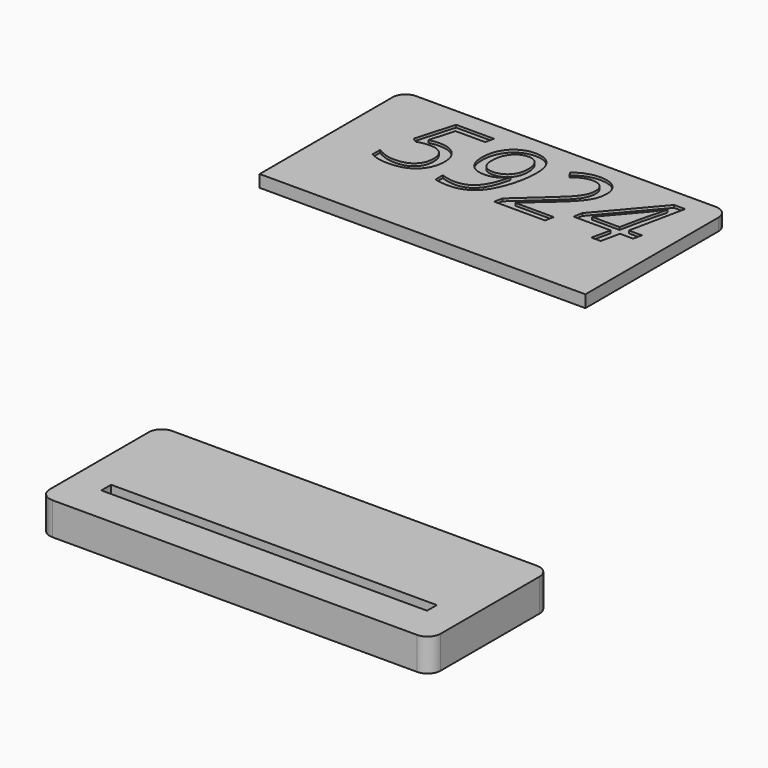
from build123d import *

# Parameters (mm, degrees)
F3_W         = 152.4
F3_H         = 58.42
F3_W_2       = 127
F3_H_2       = 4.7625
F4_DEPTH     = 12.7
F5_W         = 127
F5_H         = 4.7625
F5_W_2       = 35.6893126208
F5_H_2       = 5.08
F6_DEPTH     = 5.08
F7_R         = 5.08
F8_DEPTH     = 8.89
F9_W         = 127
F9_H         = 69.85
F10_DEPTH    = 4.7625
F9_TEXT_SIZE = 45.3111405174
F11_DEPTH    = 3.7625
F12_R        = 5.08
F13_DEPTH    = 3.302


# Not quite as in the source:
# - a length typed as a fraction of an inch, garbled in the dataset ("3 / 203.2 mm" for 3/8 in), is restored
# - a feature names something its author has since deleted; it is built from what else it names
# - Text() gives the source's letters only with a copy of the font that has no kerning and outlines rounded to 1/6400 em; it was checked with that copy


with BuildPart() as f4:
    # F3 (on Top) → F4 (new body)
    with BuildSketch(Plane.XY):
        with Locations((-9.5931086689, 18.5555488393)):
            Rectangle(F3_W, F3_H)
        with Locations((-9.5931086689, 6.0863080435)):
            Rectangle(F3_W_2, F3_H_2, mode=Mode.SUBTRACT)
    extrude(amount=F4_DEPTH)

    # F5 (on face) → F6 (cut)
    with BuildSketch(Plane(origin=(0, 0, 0), x_dir=(1, 0, 0), z_dir=(0, 0, -1))):
        Polygon((59.2411287415, -1.0063080435), (-78.4273460794, -1.0063080435), (-78.4273460794, -11.1663080435), (23.5518161207, -11.1663080435), (59.2411287415, -11.1663080435), align=None)
        with Locations((-9.5931086689, -6.0863080435)):
            Rectangle(F5_W, F5_H, mode=Mode.SUBTRACT)
        with Locations((41.3964724311, -13.7063080435)):
            Rectangle(F5_W_2, F5_H_2)
    extrude(amount=-F6_DEPTH, mode=Mode.SUBTRACT)

    # F7
    f7_edges = [f4.edges().sort_by_distance(p)[0] for p in [
        (-85.793109, -10.654451, 6.35),
        (66.606891, -10.654451, 6.35),
        (66.606891, 47.765549, 6.35),
        (-85.793109, 47.765549, 6.35),
    ]]
    fillet(f7_edges, radius=F7_R)

    # F5 (on face) → F8 (cut)
    with BuildSketch(Plane(origin=(0, 0, 0), x_dir=(1, 0, 0), z_dir=(0, 0, -1))):
        Polygon((59.2411287415, -41.7463080435), (59.2411287415, -16.2463080435), (23.5518161207, -16.2463080435), (10.8411287415, -16.2463080435), (10.8411287415, -27.1657891572), (10.8411287415, -30.3407891572), (10.8411287415, -41.7463080435), align=None)
    extrude(amount=-F8_DEPTH, mode=Mode.SUBTRACT)

    # F5 (on face) → F13 (cut)
    with BuildSketch(Plane(origin=(0, 0, 0), x_dir=(1, 0, 0), z_dir=(0, 0, -1))):
        Polygon((10.8411287415, -30.3407891572), (10.8411287415, -27.1657891572), (-11.5801747888, -27.1657891572), (-11.5801747888, -47.7655488393), (-8.4051747888, -47.7655488393), (-8.4051747888, -30.3407891572), align=None)
    extrude(amount=-F13_DEPTH, mode=Mode.SUBTRACT)


with BuildPart() as f10:
    # F9 (on Top) → F10 (new body)
    with BuildSketch(Plane.XY):
        with Locations((-111.8032857776, 243.5436563784)):
            Rectangle(F9_W, F9_H)
        with BuildLine():
            add(Edge.make_bspline(
                [(-149.1894343829, 258.2214627279), (-147.2637109109, 258.7312130587), (-145.118511602, 258.7312130587)],
                knots=[0, 0, 0, 1, 1, 1], degree=2))
            add(Edge.make_bspline(
                [(-145.118511602, 258.7312130587), (-141.0900680154, 258.7312130587), (-138.7147730711, 256.4196369058)],
                knots=[0, 0, 0, 1, 1, 1], degree=2))
            add(Edge.make_bspline(
                [(-138.7147730711, 256.4196369058), (-136.3394781268, 254.1080607528), (-136.3394781268, 250.1645755547)],
                knots=[0, 0, 0, 1, 1, 1], degree=2))
            add(Edge.make_bspline(
                [(-136.3394781268, 250.1645755547), (-136.3394781268, 246.6034031046), (-137.9536875077, 243.9059742707)],
                knots=[0, 0, 0, 1, 1, 1], degree=2))
            add(Edge.make_bspline(
                [(-137.9536875077, 243.9059742707), (-139.5678968887, 241.2085454368), (-142.4671018952, 239.8669108855)],
                knots=[0, 0, 0, 1, 1, 1], degree=2))
            add(Edge.make_bspline(
                [(-142.4671018952, 239.8669108855), (-145.3663069018, 238.5252763343), (-149.2814726371, 238.5252763343)],
                knots=[0, 0, 0, 1, 1, 1], degree=2))
            add(Edge.make_bspline(
                [(-149.2814726371, 238.5252763343), (-153.5506316577, 238.5252763343), (-156.5808141798, 240.2740031636)],
                knots=[0, 0, 0, 1, 1, 1], degree=2))
            Line((-156.5808141798, 240.2740031636), (-156.5808141798, 243.9059742707))
            add(Edge.make_bspline(
                [(-156.5808141798, 243.9059742707), (-152.9488430727, 241.6474971105), (-149.1894343829, 241.6474971105)],
                knots=[0, 0, 0, 1, 1, 1], degree=2))
            add(Edge.make_bspline(
                [(-149.1894343829, 241.6474971105), (-144.9627545565, 241.6474971105), (-142.5980794108, 243.7714568223)],
                knots=[0, 0, 0, 1, 1, 1], degree=2))
            add(Edge.make_bspline(
                [(-142.5980794108, 243.7714568223), (-140.233404265, 245.895416534), (-140.233404265, 249.7043842838)],
                knots=[0, 0, 0, 1, 1, 1], degree=2))
            add(Edge.make_bspline(
                [(-140.233404265, 249.7043842838), (-140.233404265, 252.4867715062), (-141.8582334445, 254.1151406185)],
                knots=[0, 0, 0, 1, 1, 1], degree=2))
            add(Edge.make_bspline(
                [(-141.8582334445, 254.1151406185), (-143.483062624, 255.7435097309), (-146.3787276977, 255.7435097309)],
                knots=[0, 0, 0, 1, 1, 1], degree=2))
            add(Edge.make_bspline(
                [(-146.3787276977, 255.7435097309), (-147.4407075536, 255.7435097309), (-148.5274669394, 255.5983724839)],
                knots=[0, 0, 0, 1, 1, 1], degree=2))
            add(Edge.make_bspline(
                [(-148.5274669394, 255.5983724839), (-149.6142263253, 255.4532352369), (-151.6036685886, 254.922245309)],
                knots=[0, 0, 0, 1, 1, 1], degree=2))
            Line((-151.6036685886, 254.922245309), (-153.2391175667, 256.1824614046))
            Line((-153.2391175667, 256.1824614046), (-148.8779202919, 271.3192142837))
            Line((-148.8779202919, 271.3192142837), (-134.1022405638, 271.3192142837))
            Line((-134.1022405638, 271.3192142837), (-134.8314667315, 267.9350384763))
            Line((-134.8314667315, 267.9350384763), (-146.3787276977, 267.9350384763))
            Line((-146.3787276977, 267.9350384763), (-149.1894343829, 258.2214627279))
        make_face(mode=Mode.SUBTRACT)
        with BuildLine():
            add(Edge.make_bspline(
                [(-111.9882800316, 269.2483535648), (-109.7899817299, 266.7173015749), (-109.7899817299, 261.8463539693)],
                knots=[0, 0, 0, 1, 1, 1], degree=2))
            add(Edge.make_bspline(
                [(-109.7899817299, 261.8463539693), (-109.7899817299, 257.5559553516), (-111.0289582284, 252.8549245229)],
                knots=[0, 0, 0, 1, 1, 1], degree=2))
            add(Edge.make_bspline(
                [(-111.0289582284, 252.8549245229), (-112.2679347269, 248.1538936942), (-114.289236386, 244.8900756038)],
                knots=[0, 0, 0, 1, 1, 1], degree=2))
            add(Edge.make_bspline(
                [(-114.289236386, 244.8900756038), (-116.310538045, 241.6262575134), (-119.1885034544, 240.0757669238)],
                knots=[0, 0, 0, 1, 1, 1], degree=2))
            add(Edge.make_bspline(
                [(-119.1885034544, 240.0757669238), (-122.0664688638, 238.5252763343), (-125.8683567479, 238.5252763343)],
                knots=[0, 0, 0, 1, 1, 1], degree=2))
            add(Edge.make_bspline(
                [(-125.8683567479, 238.5252763343), (-128.8772996728, 238.5252763343), (-131.2278150872, 239.2828219648)],
                knots=[0, 0, 0, 1, 1, 1], degree=2))
            Line((-131.2278150872, 239.2828219648), (-131.2278150872, 242.7802756235))
            add(Edge.make_bspline(
                [(-131.2278150872, 242.7802756235), (-128.2613513564, 241.7395353647), (-125.7833983594, 241.7395353647)],
                knots=[0, 0, 0, 1, 1, 1], degree=2))
            add(Edge.make_bspline(
                [(-125.7833983594, 241.7395353647), (-121.316003099, 241.7395353647), (-118.547775608, 244.8582162081)],
                knots=[0, 0, 0, 1, 1, 1], degree=2))
            add(Edge.make_bspline(
                [(-118.547775608, 244.8582162081), (-115.779548117, 247.9768970516), (-114.3635749759, 254.6107312179)],
                knots=[0, 0, 0, 1, 1, 1], degree=2))
            Line((-114.3635749759, 254.6107312179), (-114.5901306785, 254.6107312179))
            add(Edge.make_bspline(
                [(-114.5901306785, 254.6107312179), (-115.7158293257, 252.9540426428), (-117.5176551478, 251.9911809068)],
                knots=[0, 0, 0, 1, 1, 1], degree=2))
            add(Edge.make_bspline(
                [(-117.5176551478, 251.9911809068), (-119.31948097, 251.0283191708), (-121.5142393388, 251.0283191708)],
                knots=[0, 0, 0, 1, 1, 1], degree=2))
            add(Edge.make_bspline(
                [(-121.5142393388, 251.0283191708), (-125.2524084315, 251.0283191708), (-127.2878698219, 253.2089178082)],
                knots=[0, 0, 0, 1, 1, 1], degree=2))
            add(Edge.make_bspline(
                [(-127.2878698219, 253.2089178082), (-129.3233312123, 255.3895164456), (-129.3233312123, 259.5949566748)],
                knots=[0, 0, 0, 1, 1, 1], degree=2))
            add(Edge.make_bspline(
                [(-129.3233312123, 259.5949566748), (-129.3233312123, 262.9791324822), (-127.8967382726, 265.800458966)],
                knots=[0, 0, 0, 1, 1, 1], degree=2))
            add(Edge.make_bspline(
                [(-127.8967382726, 265.800458966), (-126.4701453329, 268.6217854498), (-123.9143138131, 270.2005955022)],
                knots=[0, 0, 0, 1, 1, 1], degree=2))
            add(Edge.make_bspline(
                [(-123.9143138131, 270.2005955022), (-121.3584822932, 271.7794055546), (-118.1725427256, 271.7794055546)],
                knots=[0, 0, 0, 1, 1, 1], degree=2))
            add(Edge.make_bspline(
                [(-118.1725427256, 271.7794055546), (-114.1865783332, 271.7794055546), (-111.9882800316, 269.2483535648)],
                knots=[0, 0, 0, 1, 1, 1], degree=2))
        make_face(mode=Mode.SUBTRACT)
        with BuildLine():
            Line((-87.6370819363, 242.3767232782), (-88.2813497155, 238.9713078737))
            Line((-88.2813497155, 238.9713078737), (-108.1686924833, 238.9713078737))
            Line((-108.1686924833, 238.9713078737), (-107.4890253755, 242.2209662327))
            Line((-107.4890253755, 242.2209662327), (-97.1949006392, 251.5168299045))
            add(Edge.make_bspline(
                [(-97.1949006392, 251.5168299045), (-94.9435033447, 253.5770708249), (-93.2938946353, 255.1346412802)],
                knots=[0, 0, 0, 1, 1, 1], degree=2))
            add(Edge.make_bspline(
                [(-93.2938946353, 255.1346412802), (-91.6442859258, 256.6922117355), (-90.5716862714, 258.0763254809)],
                knots=[0, 0, 0, 1, 1, 1], degree=2))
            add(Edge.make_bspline(
                [(-90.5716862714, 258.0763254809), (-89.4990866169, 259.4604392264), (-88.9787164876, 260.819773442)],
                knots=[0, 0, 0, 1, 1, 1], degree=2))
            add(Edge.make_bspline(
                [(-88.9787164876, 260.819773442), (-88.4583463582, 262.1791076575), (-88.4583463582, 263.8428760984)],
                knots=[0, 0, 0, 1, 1, 1], degree=2))
            add(Edge.make_bspline(
                [(-88.4583463582, 263.8428760984), (-88.4583463582, 266.0305546015), (-89.785821178, 267.3120102942)],
                knots=[0, 0, 0, 1, 1, 1], degree=2))
            add(Edge.make_bspline(
                [(-89.785821178, 267.3120102942), (-91.1132959979, 268.593465987), (-93.3930127552, 268.593465987)],
                knots=[0, 0, 0, 1, 1, 1], degree=2))
            add(Edge.make_bspline(
                [(-93.3930127552, 268.593465987), (-95.0992603903, 268.593465987), (-96.7240895698, 267.9633579392)],
                knots=[0, 0, 0, 1, 1, 1], degree=2))
            add(Edge.make_bspline(
                [(-96.7240895698, 267.9633579392), (-98.3489187493, 267.3332498913), (-100.3171214155, 265.8323183617)],
                knots=[0, 0, 0, 1, 1, 1], degree=2))
            Line((-100.3171214155, 265.8323183617), (-102.1295670362, 268.3739901501))
            add(Edge.make_bspline(
                [(-102.1295670362, 268.3739901501), (-97.9028872098, 271.7794055546), (-92.9965402756, 271.7794055546)],
                knots=[0, 0, 0, 1, 1, 1], degree=2))
            add(Edge.make_bspline(
                [(-92.9965402756, 271.7794055546), (-89.1026141374, 271.7794055546), (-86.8335171787, 269.8218226869)],
                knots=[0, 0, 0, 1, 1, 1], degree=2))
            add(Edge.make_bspline(
                [(-86.8335171787, 269.8218226869), (-84.56442022, 267.8642398193), (-84.56442022, 264.4375848176)],
                knots=[0, 0, 0, 1, 1, 1], degree=2))
            add(Edge.make_bspline(
                [(-84.56442022, 264.4375848176), (-84.56442022, 261.9808714177), (-85.4387836346, 259.9241704302)],
                knots=[0, 0, 0, 1, 1, 1], degree=2))
            add(Edge.make_bspline(
                [(-85.4387836346, 259.9241704302), (-86.3131470493, 257.8674694426), (-88.3379886412, 255.5665130882)],
                knots=[0, 0, 0, 1, 1, 1], degree=2))
            add(Edge.make_bspline(
                [(-88.3379886412, 255.5665130882), (-90.3628302331, 253.2655567338), (-94.8514650906, 249.3503909985)],
                knots=[0, 0, 0, 1, 1, 1], degree=2))
            Line((-94.8514650906, 249.3503909985), (-102.639317367, 242.5537199209))
            Line((-102.639317367, 242.5537199209), (-102.639317367, 242.3767232782))
            Line((-102.639317367, 242.3767232782), (-87.6370819363, 242.3767232782))
        make_face(mode=Mode.SUBTRACT)
        Polygon((-59.1406224703, 249.746863478), (-59.8769285037, 246.3626876706), (-65.0310707376, 246.3626876706), (-66.6240405214, 238.9713078737), (-70.2489317628, 238.9713078737), (-68.6134827847, 246.3626876706), (-83.1272074817, 246.3626876706), (-82.4829397025, 249.8601413293), (-64.032809673, 271.4962109264), (-59.6999318611, 271.4962109264), (-64.273525107, 249.746863478), align=None, mode=Mode.SUBTRACT)
    extrude(amount=F10_DEPTH)



with BuildPart() as f10b:
    # F9 (on Top) → F10, piece 2 (new body)
    with BuildSketch(Plane.XY):
        with BuildLine():
            add(Edge.make_bspline(
                [(-114.7635873882, 266.9509371432), (-116.069822611, 268.6430250469), (-118.307060174, 268.6430250469)],
                knots=[0, 0, 0, 1, 1, 1], degree=2))
            add(Edge.make_bspline(
                [(-118.307060174, 268.6430250469), (-121.6204373244, 268.6430250469), (-123.6346591177, 266.1402925199)],
                knots=[0, 0, 0, 1, 1, 1], degree=2))
            add(Edge.make_bspline(
                [(-123.6346591177, 266.1402925199), (-125.648880911, 263.6375599929), (-125.648880911, 259.7223942576)],
                knots=[0, 0, 0, 1, 1, 1], degree=2))
            add(Edge.make_bspline(
                [(-125.648880911, 259.7223942576), (-125.648880911, 256.9824862294), (-124.445303741, 255.5204939611)],
                knots=[0, 0, 0, 1, 1, 1], degree=2))
            add(Edge.make_bspline(
                [(-124.445303741, 255.5204939611), (-123.241726571, 254.0585016929), (-120.8487319624, 254.0585016929)],
                knots=[0, 0, 0, 1, 1, 1], degree=2))
            add(Edge.make_bspline(
                [(-120.8487319624, 254.0585016929), (-119.1708037901, 254.0585016929), (-117.754830649, 254.6886097407)],
                knots=[0, 0, 0, 1, 1, 1], degree=2))
            add(Edge.make_bspline(
                [(-117.754830649, 254.6886097407), (-116.3388575078, 255.3187177885), (-115.3512162418, 256.4939754957)],
                knots=[0, 0, 0, 1, 1, 1], degree=2))
            add(Edge.make_bspline(
                [(-115.3512162418, 256.4939754957), (-114.3635749759, 257.6692332029), (-113.9104635707, 259.0179476198)],
                knots=[0, 0, 0, 1, 1, 1], degree=2))
            add(Edge.make_bspline(
                [(-113.9104635707, 259.0179476198), (-113.4573521655, 260.3666620368), (-113.4573521655, 262.3561043001)],
                knots=[0, 0, 0, 1, 1, 1], degree=2))
            add(Edge.make_bspline(
                [(-113.4573521655, 262.3561043001), (-113.4573521655, 265.2588492395), (-114.7635873882, 266.9509371432)],
                knots=[0, 0, 0, 1, 1, 1], degree=2))
        make_face()
    extrude(amount=F10_DEPTH)


with BuildPart() as f10c:
    # F9 (on Top) → F10, piece 3 (new body)
    with BuildSketch(Plane.XY):
        with BuildLine():
            Line((-78.6385726242, 249.746863478), (-67.884256617, 249.746863478))
            add(Edge.make_bspline(
                [(-67.884256617, 249.746863478), (-66.8647559554, 254.6107312179), (-66.1567693848, 257.9984469582)],
                knots=[0, 0, 0, 1, 1, 1], degree=2))
            add(Edge.make_bspline(
                [(-66.1567693848, 257.9984469582), (-65.4487828142, 261.3861626984), (-63.5938579993, 267.8430002222)],
                knots=[0, 0, 0, 1, 1, 1], degree=2))
            Line((-63.5938579993, 267.8430002222), (-63.7708546419, 267.8430002222))
            add(Edge.make_bspline(
                [(-63.7708546419, 267.8430002222), (-64.1460875243, 267.2058123086), (-65.2399267759, 265.7119606447)],
                knots=[0, 0, 0, 1, 1, 1], degree=2))
            add(Edge.make_bspline(
                [(-65.2399267759, 265.7119606447), (-66.3337660274, 264.2181089808), (-66.8435163583, 263.5738412015)],
                knots=[0, 0, 0, 1, 1, 1], degree=2))
            Line((-66.8435163583, 263.5738412015), (-78.6385726242, 249.746863478))
        make_face()
    extrude(amount=F10_DEPTH)


with BuildPart() as f10_1:
    add(f10.part)

    add(f10b.part)  # F11 merges F10b

    add(f10c.part)  # F11 merges F10c
    # F9 (on Top) → F11 (join)
    with BuildSketch(Plane.XY):
        with Locations((-158.3507806063, 238.9713078737)):
            Text('5924', F9_TEXT_SIZE, font='Open Sans', font_style=FontStyle.ITALIC, text_align=(TextAlign.LEFT, TextAlign.BOTTOM))
    extrude(amount=F11_DEPTH)

    # F12
    f12_edges = [f10_1.edges().sort_by_distance(p)[0] for p in [
        (-175.303286, 278.468656, 2.38125),
        (-48.303286, 278.468656, 2.38125),
    ]]
    fillet(f12_edges, radius=F12_R)


solid = Compound([f4.part, f10_1.part])
